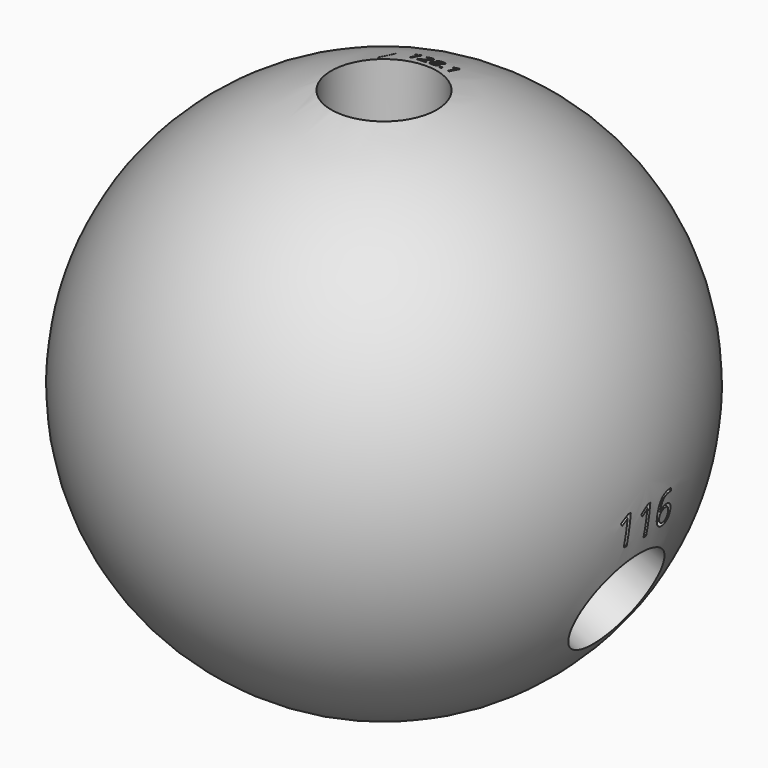
from build123d import *

# Parameters (mm, degrees)
F4_R          = 3.175
F5_DEPTH      = 25.4
F7_TEXT_SIZE  = 1.1479682548
F8_DEPTH      = 10.16
F10_ANGLE     = 116
F12_TEXT_SIZE = 1.5955812867
F13_DEPTH     = 10.16
F15_ANGLE     = -116
F17_TEXT_SIZE = 2.4789045306
F18_DEPTH     = 10.16


# Not quite as in the source:
# - Text() gives the source's letters only with a copy of the font that has no kerning and outlines rounded to 1/6400 em; it was checked with that copy


with BuildPart() as f2:
    # F0 (on Front) → F2 (revolve)
    with BuildSketch(Plane.XZ):
        with BuildLine():
            Line((15.875, 0), (-15.875, 0))
            ThreePointArc((-15.875, 0), (0, -15.875), (15.875, 0))
        make_face()
    revolve(axis=Axis((0, 0, 0), (1, 0, 0)))

    # F7 (on offset) → F8 (cut)
    with BuildSketch(Plane.XY.offset(19.05)):
        with Locations((-1.6372704413, 3.6113988608)):
            Text('128.1', F7_TEXT_SIZE, font='Open Sans', text_align=(TextAlign.LEFT, TextAlign.BOTTOM))
    extrude(amount=-F8_DEPTH, mode=Mode.SUBTRACT)

    # F12 (on offset) → F13 (cut)
    with BuildSketch(Plane(origin=(-17.122026582, 0, -8.3509703463), x_dir=(0, -1, 0), z_dir=(-0.8987940463, 0, -0.4383711468))):
        with Locations((-1.4439370134, 3.4726131707)):
            Text('116', F12_TEXT_SIZE, font='Open Sans', text_align=(TextAlign.LEFT, TextAlign.BOTTOM))
    extrude(amount=-F13_DEPTH, mode=Mode.SUBTRACT)

    # F17 (on offset) → F18 (cut)
    with BuildSketch(Plane(origin=(17.122026582, 0, -8.3509703463), x_dir=(0, 1, 0), z_dir=(0.8987940463, 0, -0.4383711468))):
        with Locations((-2.0398683846, 4.0550907142)):
            Text('116', F17_TEXT_SIZE, font='Open Sans', text_align=(TextAlign.LEFT, TextAlign.BOTTOM))
    extrude(amount=-F18_DEPTH, mode=Mode.SUBTRACT)


with BuildPart() as f5:
    # F4 (on offset) → F5 (new body)
    with BuildSketch(Plane.XY.offset(6.35)):
        Circle(F4_R)
    extrude(amount=F5_DEPTH)


with BuildPart() as f10_1:
    # F10: copy of F5
    add(f5.part.rotate(Axis((0, 14.7483889014, 0), (0, -1, 0)), F10_ANGLE))


with BuildPart() as f15_1:
    # F15: copy of F5
    add(f5.part.rotate(Axis((0, 17.6980663091, 0), (0, -1, 0)), F15_ANGLE))


with BuildPart() as f2_1:
    add(f2.part)

    # F19: cut F5, F15_1, F10_1
    add(f5.part, mode=Mode.SUBTRACT)
    add(f15_1.part, mode=Mode.SUBTRACT)
    add(f10_1.part, mode=Mode.SUBTRACT)


solid = f2_1.part
